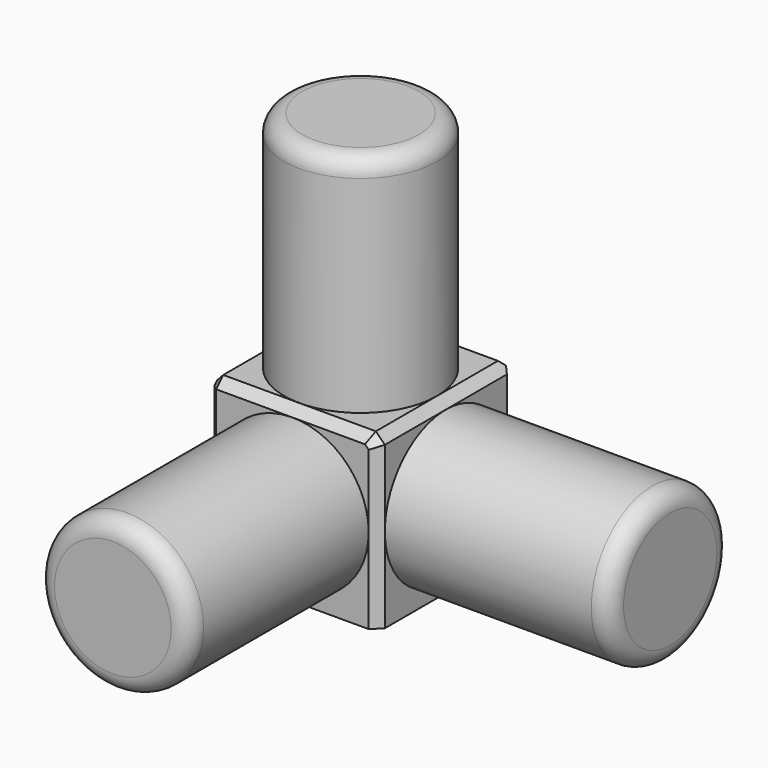
from build123d import *

# Parameters (mm, degrees)
F0_W     = 19
F0_H     = 19
F1_DEPTH = 19
F2_R     = 8.5
F5_DEPTH = 25
F3_R     = 8.5
F6_DEPTH = 25
F4_R     = 8.5
F7_DEPTH = 25
F8_R     = 2
F9_R     = 7
F10_SIZE = 0.99999
F11_SIZE = 0.99999
F12_SIZE = 0.99999


# Not quite as in the source:
# - a fillet or chamfer is up to 0.001 mm smaller than in the source, because OpenCascade refuses the exact size


with BuildPart() as f1:
    # F0 (on Top) → F1 (new body)
    with BuildSketch(Plane.XY):
        with Locations((-4.8786746205, -4.1296786368)):
            Rectangle(F0_W, F0_H)
    extrude(amount=F1_DEPTH)

    # F2 (on face) → F5 (join)
    with BuildSketch(Plane.XZ.offset(13.6296786368)):
        with Locations((-4.8786746205, 9.5)):
            Circle(F2_R)
    extrude(amount=F5_DEPTH)

    # F3 (on face) → F6 (join)
    with BuildSketch(Plane.YZ.offset(4.6213253795)):
        with Locations((-4.1296786368, 9.5)):
            Circle(F3_R)
    extrude(amount=F6_DEPTH)

    # F4 (on face) → F7 (join)
    with BuildSketch(Plane.XY.offset(19)):
        with Locations((-4.8786746205, -4.1296786368)):
            Circle(F4_R)
    extrude(amount=F7_DEPTH)

    # F8
    f8_edges = [f1.edges().sort_by_distance(p)[0] for p in [
        (-13.378675, -38.629679, 9.5),
        (29.621325, -12.629679, 9.5),
        (-13.378675, -4.129679, 44),
    ]]
    fillet(f8_edges, radius=F8_R)

    # F9
    f9_edges = [f1.edges().sort_by_distance(p)[0] for p in [
        (-14.378675, 5.370321, 9.5),
    ]]
    fillet(f9_edges, radius=F9_R)

    # F10 (size 1 in the source; OpenCascade refuses exactly that, so slightly less here)
    f10_edges = [f1.edges().sort_by_distance(p)[0] for p in [
        (4.621325, -4.129679, 19),
    ]]
    chamfer(f10_edges, length=F10_SIZE)

    # F11 (size 1 in the source; OpenCascade refuses exactly that, so slightly less here)
    f11_edges = [f1.edges().sort_by_distance(p)[0] for p in [
        (4.621325, -13.629679, 9.000005),
        (4.12133, -13.629679, 18.500005),
        (-5.37867, -13.629679, 19),
    ]]
    chamfer(f11_edges, length=F11_SIZE)

    # F12 (call 1 of 2: OpenCascade refuses the feature's edges together) (size 1 in the source; OpenCascade refuses exactly that, so slightly less here)
    f12_edges = [f1.edges().sort_by_distance(p)[0] for p in [
        (-1.87867, 5.370321, 19),
        (-12.328422, 3.320069, 19),
        (-14.378675, -7.129684, 19),
        (-14.378675, -13.629679, 9.000005),
        (-14.378675, -13.129684, 18.500005),
    ]]
    chamfer(f12_edges, length=F12_SIZE)

    # F12#2 (call 2 of 2) (size 1 in the source; OpenCascade refuses exactly that, so slightly less here)
    f12_2_edges = [f1.edges().sort_by_distance(p)[0] for p in [
        (4.621325, 5.370321, 9.000005),
    ]]
    chamfer(f12_2_edges, length=F12_SIZE)


solid = f1.part
